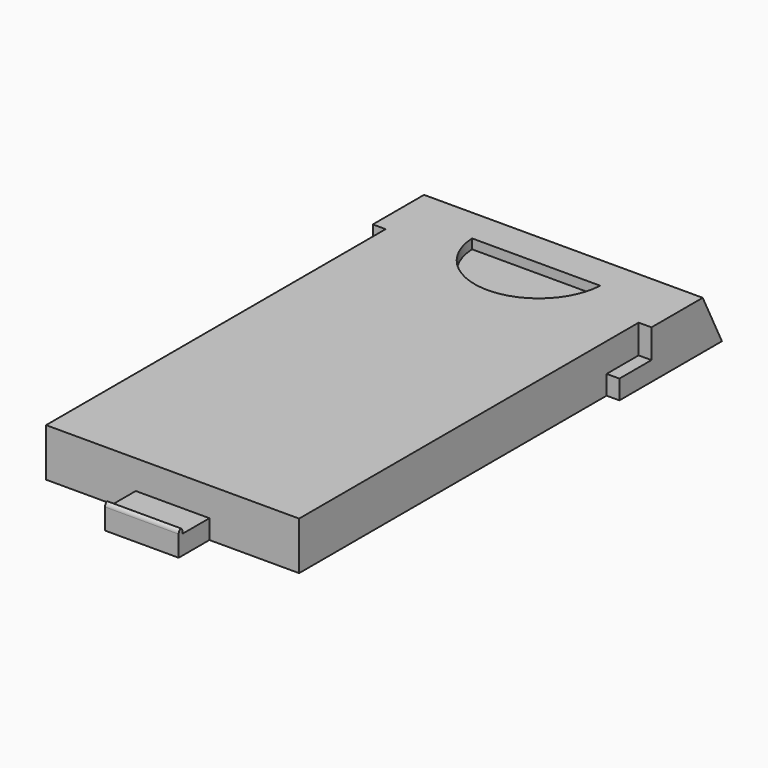
from build123d import *

# Parameters (mm, degrees)
F0_W         = 15.8
F0_H         = 32
F1_DEPTH     = 3
F3_DEPTH     = 0.8
F5_W         = 4.6
F5_H         = 1.2
F6_DEPTH     = 2.4
F8_DEPTH     = 0.6
F9_W         = 4.6
F9_H         = 0.3
F10_DEPTH    = 0.4
F11_T1_DEPTH = 6.1
F12_SIZE2    = 1.49999
F12_SIZE     = 2.99999


# Not quite as in the source:
# - a fillet or chamfer that OpenCascade refuses, or shapes differently, is made with other operations: its cross-section is extruded or revolved along the edge and cut away or added
# - a fillet or chamfer is up to 0.001 mm smaller than in the source, because OpenCascade refuses the exact size


with BuildPart() as f1:
    # F0 (on Top) → F1 (new body)
    with BuildSketch(Plane.XY):
        with Locations((0, -4.9953348935)):
            Rectangle(F0_W, F0_H)
    extrude(amount=F1_DEPTH)

    # F2 (on face) → F3 (join)
    with BuildSketch(Plane.YZ.offset(7.9)):
        Polygon((11.0046651065, 0), (11.0046651065, 3), (5.5046651065, 3), (5.5046651065, 1.2), (3.0046651065, 1.2), (3.0046651065, 0), align=None)
    extrude(amount=F3_DEPTH)

    # F4: F1 across plane


with BuildPart() as f1_1:
    add(f1.part)
    add(f1.part.mirror(Plane.YZ))

    # F5 (on face) → F6 (join)
    with BuildSketch(Plane.XZ.offset(20.9953348935)):
        with Locations((0, 0.6)):
            Rectangle(F5_W, F5_H)
    extrude(amount=F6_DEPTH)

    # F7 (on face) → F8 (cut)
    with BuildSketch(Plane.XY.offset(3)):
        with BuildLine():
            Line((4, 7.3774643242), (-4, 7.3774643242))
            ThreePointArc((-4, 7.3774643242), (0, 3.5808500116), (4, 7.3774643242))
        make_face()
    extrude(amount=-F8_DEPTH, mode=Mode.SUBTRACT)

    # F9 (on face) → F10 (join)
    with BuildSketch(Plane.XY.offset(1.2)):
        with Locations((0, -23.2453348935)):
            Rectangle(F9_W, F9_H)
    extrude(amount=F10_DEPTH)

    # F11: fillet of radius 0.3 on 2 edges, made by hand

    # F11_s2 → F11_t1 (cut)
    with BuildSketch(Plane.YZ.offset(-3.05)):
        with BuildLine():
            ThreePointArc((-23.0953348935, 1.6), (-23.3074669278, 1.5121320344), (-23.3953348935, 1.3))
            Line((-23.3953348935, 1.3), (-23.3953348935, 1.6))
            Line((-23.3953348935, 1.6), (-23.0953348935, 1.6))
        make_face()
        with BuildLine():
            ThreePointArc((-23.0953348935, 1.3), (-23.1832028591, 1.5121320344), (-23.3953348935, 1.6))
            Line((-23.3953348935, 1.6), (-23.0953348935, 1.6))
            Line((-23.0953348935, 1.6), (-23.0953348935, 1.3))
        make_face()
    extrude(amount=F11_T1_DEPTH, mode=Mode.SUBTRACT)

    # F12 (size 3 and 1.5 in the source; OpenCascade refuses exactly that, so slightly less here)
    f12_edges = [f1_1.edges().sort_by_distance(p)[0] for p in [
        (0, 11.004665, 3),
    ]]
    chamfer(f12_edges, length=F12_SIZE, length2=F12_SIZE2)


solid = f1_1.part
